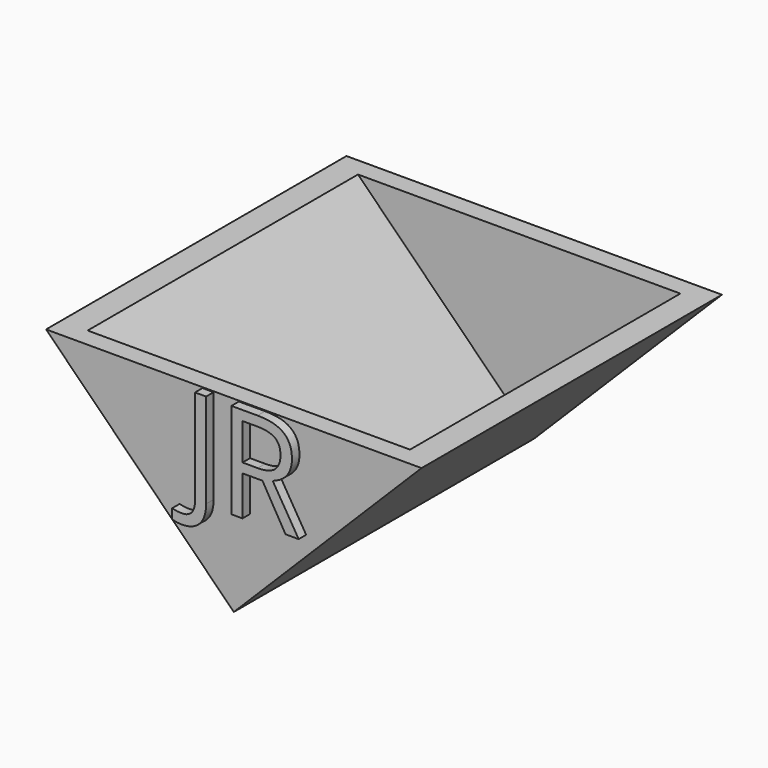
from build123d import *

# Parameters (mm, degrees)
F1_DEPTH     = 50.8
F2_T         = -2.54
F3_TEXT_SIZE = 18.0893997851
F4_DEPTH     = 1.27


# Not quite as in the source:
# - Text() gives the source's letters only with a copy of the font that has no kerning and outlines rounded to 1/6400 em; it was checked with that copy


with BuildPart() as f1:
    # F0 (on Front) → F1 (new body)
    with BuildSketch(Plane.XZ):
        Polygon((25.4, -5.8822329104), (-25.4, -5.8822329104), (0, -31.2822329104), align=None)
    extrude(amount=F1_DEPTH)

    # F2
    f2_openings = [f1.faces().sort_by_distance(p)[0] for p in [
        (0, -25.4, -5.882233),
    ]]
    offset(amount=F2_T, openings=f2_openings)

    # F3 (on face) → F4 (join)
    with BuildSketch(Plane.XZ.offset(50.8)):
        with Locations((-5.9144469092, -18.9066007556)):
            Text('JR', F3_TEXT_SIZE, font='Open Sans', text_align=(TextAlign.LEFT, TextAlign.BOTTOM))
    extrude(amount=F4_DEPTH)


solid = f1.part
